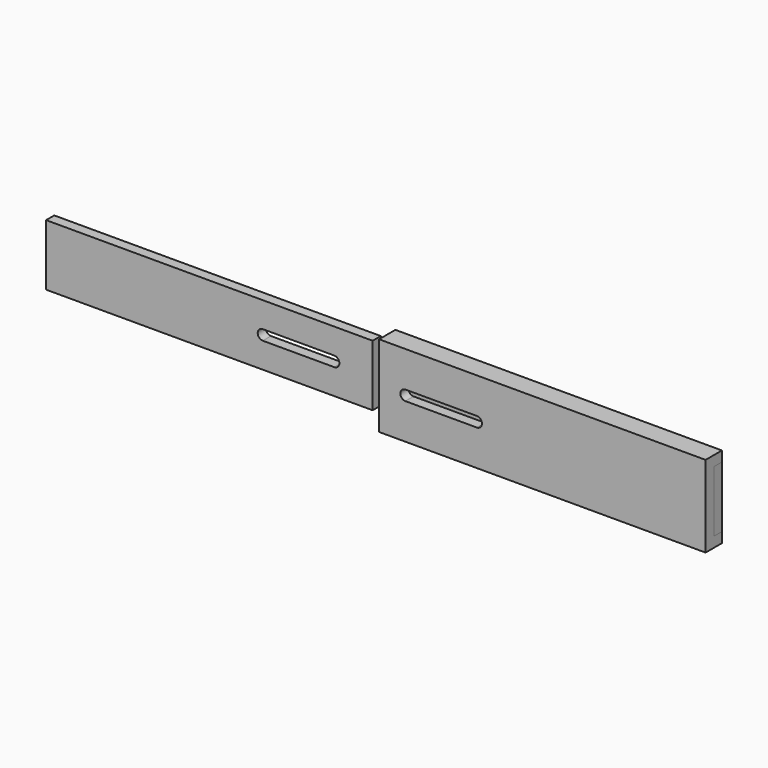
from build123d import *

# Parameters (mm, degrees)
F0_W     = 101.6
F0_H     = 19.05
F1_DEPTH = 3.175
F4_DEPTH = 101.6
F5_W     = 22.225
F5_H     = 3.175
F6_DEPTH = 3.176
F7_W     = 22.225
F7_H     = 3.175
F8_DEPTH = 25.4


with BuildPart() as f1:
    # F0 (on Front) → F1 (new body)
    with BuildSketch(Plane.XZ):
        with Locations((-50.8, 0)):
            Rectangle(F0_W, F0_H)
    extrude(amount=F1_DEPTH)


with BuildPart() as f2_1:
    # F2: copy of F1
    add(f1.part.moved(Location((106.14878, 0, 0))))


with BuildPart() as f4:
    # F3 (on face) → F4 (new body, through all)
    with BuildSketch(Plane.YZ.offset(106.14878)):
        Polygon((0, -12.7), (0, -9.525), (-3.175, -9.525), (-3.175, 9.525), (0, 9.525), (0, 12.7), (-6.35, 12.7), (-6.35, -12.7), align=None)
    extrude(amount=-F4_DEPTH)

    # F7 (on face) → F8 (cut)
    with BuildSketch(Plane.XZ.offset(6.35)):
        with Locations((23.8581371099, 0)):
            Rectangle(F7_W, F7_H)
        with BuildLine():
            Line((12.7456371099, -1.5875), (12.7456371099, 1.5875))
            ThreePointArc((12.7456371099, 1.5875), (11.1581371099, 0), (12.7456371099, -1.5875))
        make_face()
        with BuildLine():
            ThreePointArc((34.9706371099, -1.5875), (36.5581371099, 0), (34.9706371099, 1.5875))
            Line((34.9706371099, 1.5875), (34.9706371099, -1.5875))
        make_face()
    extrude(amount=-F8_DEPTH, mode=Mode.SUBTRACT)


with BuildPart() as f1_1:
    add(f1.part)

    # F5 (on face) → F6 (cut, through all)
    with BuildSketch(Plane.XZ.offset(3.175)):
        with Locations((-23.0465307151, 0)):
            Rectangle(F5_W, F5_H)
        with BuildLine():
            Line((-34.1590307151, -1.5875), (-34.1590307151, 1.5875))
            ThreePointArc((-34.1590307151, 1.5875), (-35.7465307151, 0), (-34.1590307151, -1.5875))
        make_face()
        with BuildLine():
            ThreePointArc((-11.9340307151, -1.5875), (-10.3465307151, 0), (-11.9340307151, 1.5875))
            Line((-11.9340307151, 1.5875), (-11.9340307151, -1.5875))
        make_face()
    extrude(amount=-F6_DEPTH, mode=Mode.SUBTRACT)


solid = Compound([f2_1.part, f4.part, f1_1.part])
